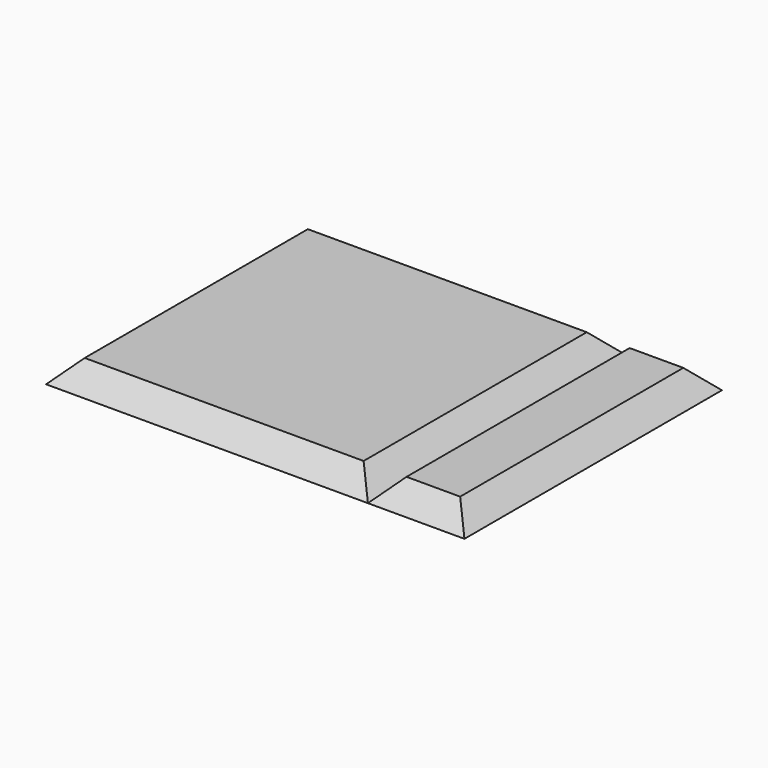
from build123d import *

# Parameters (mm, degrees)
F0_W     = 300
F0_H     = 300
F1_DEPTH = 20
F2_SIZE  = 19.99999
F3_W     = 90
F3_H     = 300
F4_DEPTH = 20
F5_SIZE  = 19.99999


# Not quite as in the source:
# - a fillet or chamfer is up to 0.001 mm smaller than in the source, because OpenCascade refuses the exact size


with BuildPart() as f1:
    # F0 (on Top) → F1 (new body)
    with BuildSketch(Plane.XY):
        with Locations((-150, 150)):
            Rectangle(F0_W, F0_H)
    extrude(amount=F1_DEPTH)

    # F2 (size 20 in the source; OpenCascade refuses exactly that, so slightly less here)
    f2_edges = [f1.edges().sort_by_distance(p)[0] for p in [
        (-150, 0, 20),
        (0, 150, 20),
        (-150, 300, 20),
        (-300, 150, 20),
    ]]
    chamfer(f2_edges, length=F2_SIZE)


with BuildPart() as f4:
    # F3 (on Top) → F4 (new body)
    with BuildSketch(Plane.XY):
        with Locations((45, 150)):
            Rectangle(F3_W, F3_H)
    extrude(amount=F4_DEPTH)

    # F5 (size 20 in the source; OpenCascade refuses exactly that, so slightly less here)
    f5_edges = [f4.edges().sort_by_distance(p)[0] for p in [
        (0, 150, 20),
        (45, 0, 20),
        (90, 150, 20),
        (45, 300, 20),
    ]]
    chamfer(f5_edges, length=F5_SIZE)


solid = Compound([f1.part, f4.part])
